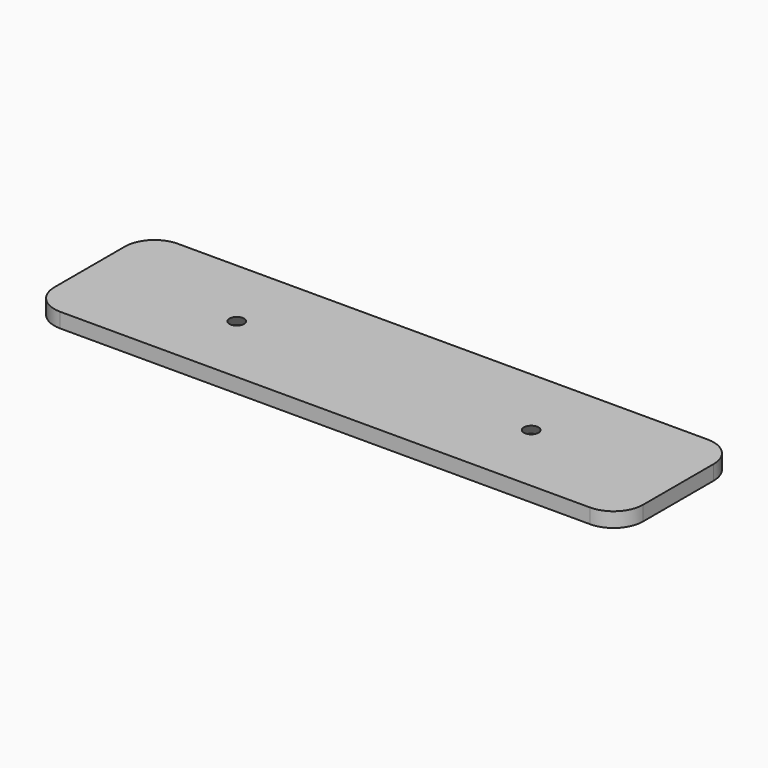
from build123d import *

# Parameters (mm, degrees)
F0_R     = 2.5
F1_DEPTH = 5
F2_SIZE  = 4.99999


# Not quite as in the source:
# - a fillet or chamfer is up to 0.001 mm smaller than in the source, because OpenCascade refuses the exact size


with BuildPart() as f1:
    # F0 (on Top) → F1 (new body)
    with BuildSketch(Plane.XY):
        with BuildLine():
            ThreePointArc((100, 15), (97.0710678119, 22.0710678119), (90, 25))
            Line((90, 25), (-90, 25))
            ThreePointArc((-90, 25), (-97.0710678119, 22.0710678119), (-100, 15))
            Line((-100, 15), (-100, -15))
            ThreePointArc((-100, -15), (-97.0710678119, -22.0710678119), (-90, -25))
            Line((-90, -25), (90, -25))
            ThreePointArc((90, -25), (97.0710678119, -22.0710678119), (100, -15))
            Line((100, -15), (100, 15))
        make_face()
        with Locations((-50, 0)):
            Circle(F0_R, mode=Mode.SUBTRACT)
        with Locations((50, 0)):
            Circle(F0_R, mode=Mode.SUBTRACT)
    extrude(amount=F1_DEPTH)

    # F2 (size 5 in the source; OpenCascade refuses exactly that, so slightly less here)
    f2_edges = [f1.edges().sort_by_distance(p)[0] for p in [
        (-52.5, 0, 0),
        (47.5, 0, 0),
    ]]
    chamfer(f2_edges, length=F2_SIZE)


solid = f1.part
